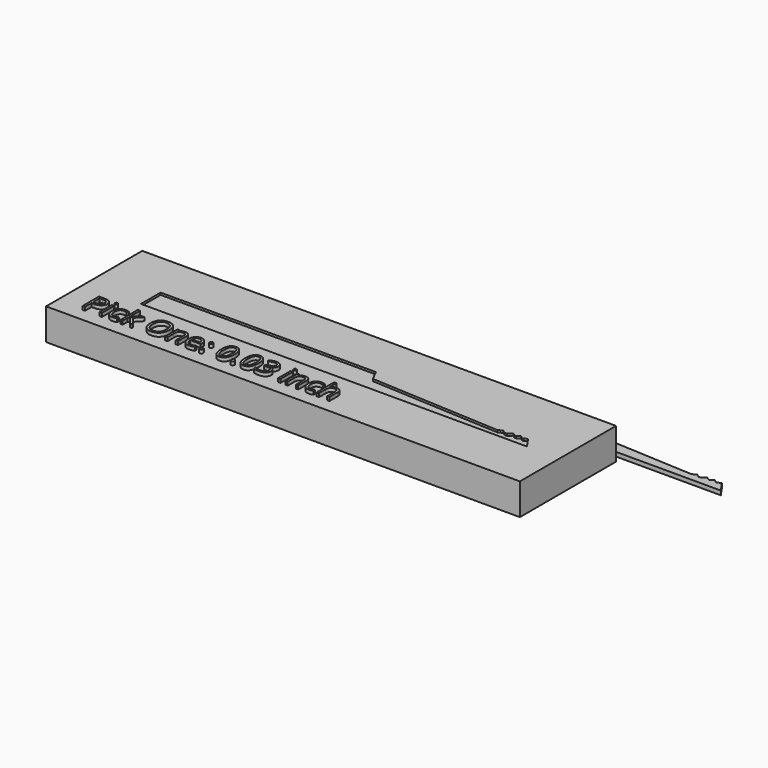
from build123d import *

# Parameters (mm, degrees)
F1_DEPTH     = 1.524
F2_W         = 182.5792118907
F2_H         = 43.6144741252
F3_DEPTH     = 25.4
F5_DEPTH     = 33.782
F4_W         = 13.7265171131
F4_H         = 8.9278469177
F6_DEPTH     = 0.762
F7_DEPTH     = 44.45
F8_DEPTH     = 13.97
F9_TEXT_SIZE = 10.3948405012
F10_DEPTH    = 1.27


# Not quite as in the source:
# - Text() gives the source's letters only with a copy of the font that has no kerning and outlines rounded to 1/6400 em; it was checked with that copy


with BuildPart() as f1:
    # F0 (on Top) → F1 (new body)
    with BuildSketch(Plane.XY):
        Polygon((-80.01, 41.4695973172), (-80.01, 32.5417503995), (0, 32.5417503995), (60.0296942423, 32.5417503995), (57.3306256048, 36.4286201875), (56.2628505302, 35.6871499627), (55.7719905529, 35.6871499627), (54.7906256048, 36.4286201875), (53.6061288199, 35.6626132912), (53.0288587161, 35.6626132912), (51.9966256048, 36.4425169536), (50.6295181289, 35.2007957653), (49.7636081635, 35.2007957653), (48.6946256048, 36.0084654703), (47.2236081635, 35.2007957653), (0, 37.6974442349), (-0.7566144174, 39.1956412988), (-1.905, 41.4695973172), align=None)
    extrude(amount=F1_DEPTH)


with BuildPart() as f3:
    # F2 (on Top) → F3 (new body)
    with BuildSketch(Plane.XY):
        with Locations((-6.1160512269, -12.6331574284)):
            Rectangle(F2_W, F2_H)
    extrude(amount=F3_DEPTH)

    # F5 (add): a face of the model
    f5_faces = [f3.faces().sort_by_distance(p)[0] for p in [
        (-97.4056571722, -12.6331574284, 12.7),
    ]]
    extrude(f5_faces, amount=F5_DEPTH)

    # F4 (on face) → F6 (cut)
    with BuildSketch(Plane.XY.offset(25.4)):
        Polygon((-97.4056571722, -7.5530489152), (-97.4056571722, -16.4808958329), (-31.1221742853, -16.4808958329), (28.907519957, -16.4808958329), (26.2084513195, -12.5940260449), (25.1406762449, -13.3354962697), (24.6498162676, -13.3354962697), (23.6684513195, -12.5940260449), (22.4839545346, -13.3600329412), (21.9066844308, -13.3600329412), (20.8744513195, -12.5801292789), (19.5073438436, -13.8218504672), (18.6414338782, -13.8218504672), (17.5724513195, -13.0141807621), (16.1014338782, -13.8218504672), (-31.1221742853, -11.3252019975), (-31.8787887027, -9.8270049336), (-33.0271742853, -7.5530489152), align=None)
        with Locations((-104.2689157288, -12.016972374)):
            Rectangle(F4_W, F4_H)
    extrude(amount=-F6_DEPTH, mode=Mode.SUBTRACT)

    # F7 (cut): a face of the model
    f7_faces = [f3.faces().sort_by_distance(p)[0] for p in [
        (85.1735547185, -12.6331574284, 12.7),
    ]]
    extrude(f7_faces, amount=-F7_DEPTH, mode=Mode.SUBTRACT)

    # F8 (cut): a face of the model
    f8_faces = [f3.faces().sort_by_distance(p)[0] for p in [
        (-45.2320512269, -12.6331574284, 0),
    ]]
    extrude(f8_faces, amount=-F8_DEPTH, mode=Mode.SUBTRACT)

    # F9 (on face) → F10 (join)
    with BuildSketch(Plane.XY.offset(25.4)):
        with Locations((-122.7574646473, -29.6667795628)):
            Text('Pick One: 0.03 inch', F9_TEXT_SIZE, font='Open Sans', text_align=(TextAlign.LEFT, TextAlign.BOTTOM))
    extrude(amount=F10_DEPTH)


solid = Compound([f1.part, f3.part])
